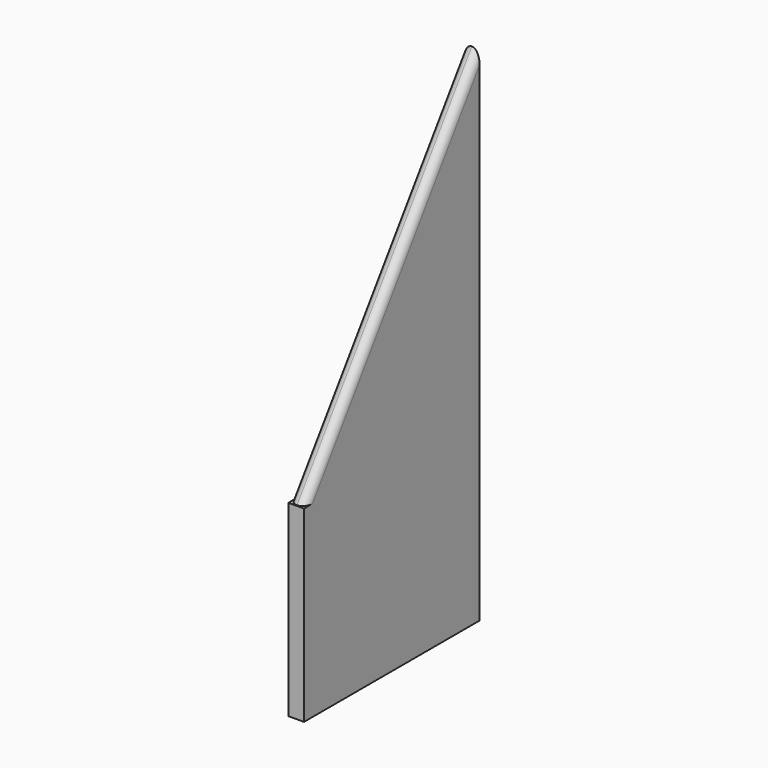
from build123d import *

# Parameters (mm, degrees)
F0_W     = 0.6239625519
F0_H     = 120
F1_DEPTH = 10
F2_R     = 4.99999


# Not quite as in the source:
# - a fillet or chamfer is up to 0.001 mm smaller than in the source, because OpenCascade refuses the exact size


with BuildPart() as f1:
    # F0 (on Right) → F1 (new body)
    with BuildSketch(Plane.YZ):
        with Locations((-139.943079155, 60)):
            Rectangle(F0_W, F0_H)
        Polygon((-139.631097879, 120), (-139.631097879, 0), (0, 0), (0, 321.3160612199), align=None)
    extrude(amount=F1_DEPTH)

    # F2 (radius 5 in the source; OpenCascade refuses exactly that, so slightly less here)
    f2_edges = [f1.edges().sort_by_distance(p)[0] for p in [
        (10, -69.815549, 220.658031),
        (0, -69.815549, 220.658031),
    ]]
    fillet(f2_edges, radius=F2_R)


solid = f1.part
